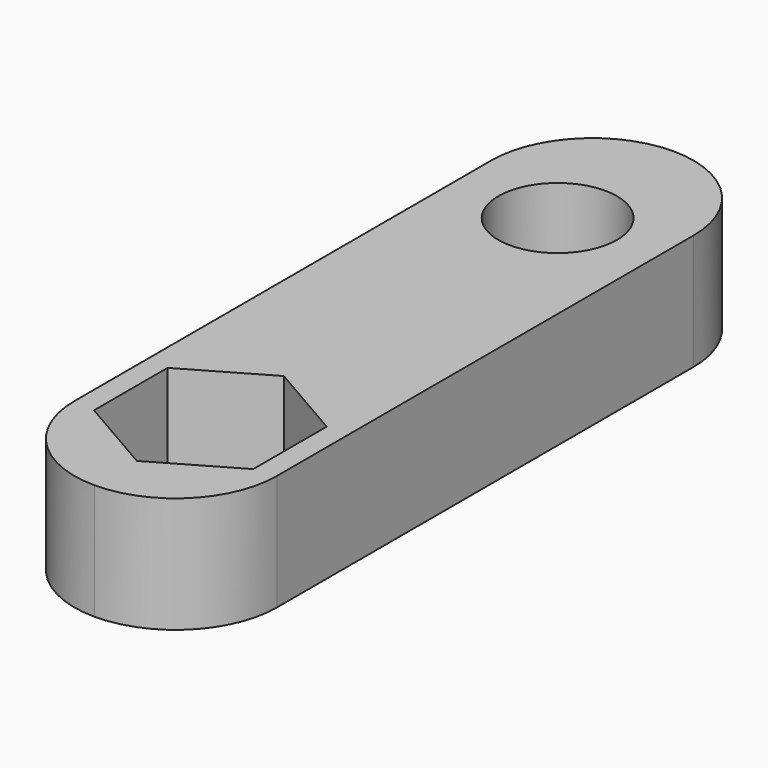
from build123d import *

# Parameters (mm, degrees)
F0_R     = 2.05
F1_DEPTH = 1
F2_DEPTH = 3
F3_R     = 3.49999


# Not quite as in the source:
# - a fillet or chamfer is up to 0.001 mm smaller than in the source, because OpenCascade refuses the exact size


with BuildPart() as f1:
    # F0 (on Top) → F1 (new body)
    with BuildSketch(Plane.XY):
        Polygon((-3.5, -20), (3.5, -20), (3.5, 5), (0, 5), (-3.5, 5), align=None)
        Polygon((0, -18.1754264805), (-2.75, -16.5877132403), (-2.75, -13.4122867597), (0, -11.8245735195), (2.75, -13.4122867597), (2.75, -16.5877132403), align=None, mode=Mode.SUBTRACT)
        Circle(F0_R, mode=Mode.SUBTRACT)
        Polygon((-2.75, -13.4122867597), (-2.75, -16.5877132403), (0, -18.1754264805), (2.75, -16.5877132403), (2.75, -13.4122867597), (0, -11.8245735195), align=None)
    extrude(amount=-F1_DEPTH)

    # F0 (on Top) → F2 (join)
    with BuildSketch(Plane.XY):
        Polygon((-3.5, -20), (3.5, -20), (3.5, 5), (0, 5), (-3.5, 5), align=None)
        Polygon((0, -18.1754264805), (-2.75, -16.5877132403), (-2.75, -13.4122867597), (0, -11.8245735195), (2.75, -13.4122867597), (2.75, -16.5877132403), align=None, mode=Mode.SUBTRACT)
        Circle(F0_R, mode=Mode.SUBTRACT)
    extrude(amount=F2_DEPTH)

    # F3 (radius 3.5 in the source; OpenCascade refuses exactly that, so slightly less here)
    f3_edges = [f1.edges().sort_by_distance(p)[0] for p in [
        (3.5, -20, 1),
        (-3.5, -20, 1),
        (3.5, 5, 1),
        (-3.5, 5, 1),
    ]]
    fillet(f3_edges, radius=F3_R)


solid = f1.part
